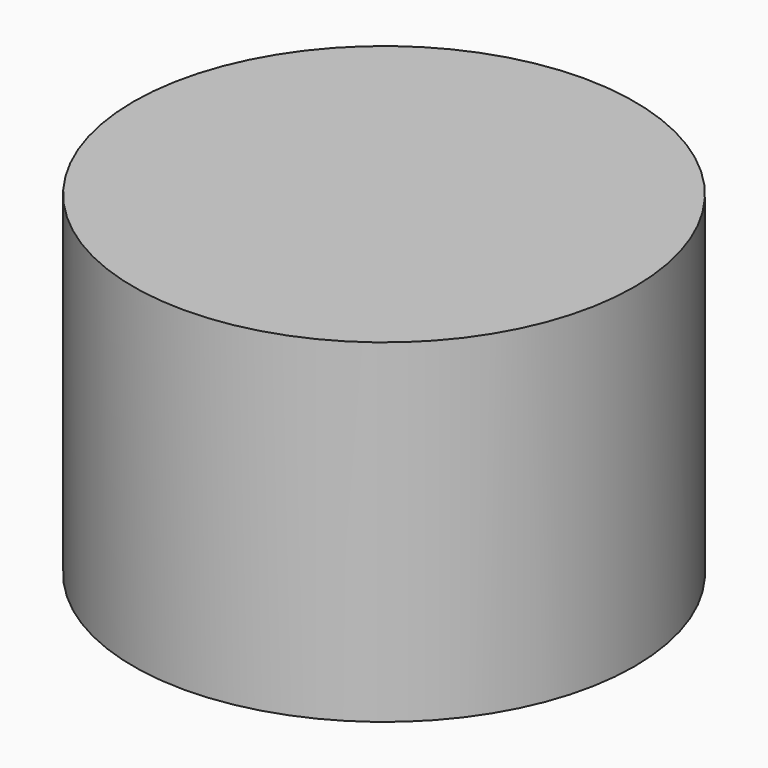
from build123d import *

# Parameters (mm, degrees)
F0_R     = 38.1
F1_DEPTH = 50.8


# Not quite as in the source:
# - a feature of the source that left no trace in its solid (it failed there, or was rolled back) is left out
# - the program builds the solid bodies; features that only make, move or delete a surface that nothing else refers to are left out


with BuildPart() as f1:
    # F0 (on Top) → F1 (new body)
    with BuildSketch(Plane.XY):
        Circle(F0_R)
    extrude(amount=F1_DEPTH)


solid = f1.part
